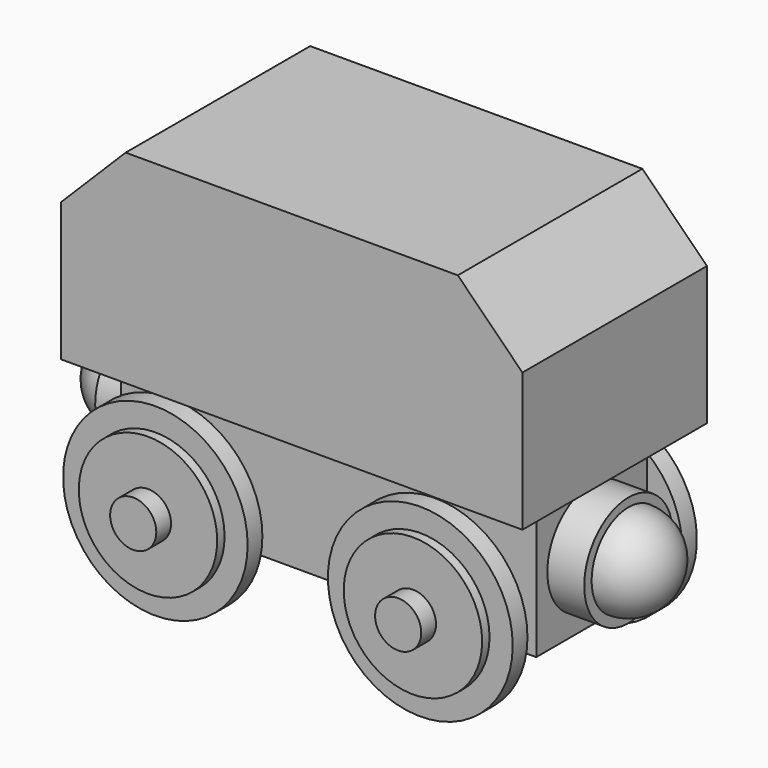
from build123d import *

# Parameters (mm, degrees)
F0_W      = 50
F0_H      = 22
F1_DEPTH  = 12.5
F2_W      = 45
F2_H      = 15
F3_DEPTH  = 15
F4_R      = 2.5
F5_DEPTH  = 3
F6_R      = 2.5
F7_DEPTH  = 3
F8_R      = 2.5
F9_DEPTH  = 3
F10_R     = 2.5
F11_DEPTH = 3
F12_R     = 10
F13_DEPTH = 2
F14_R     = 10
F15_DEPTH = 2
F16_R     = 10
F17_DEPTH = 2
F18_R     = 10.0146932226
F19_DEPTH = 2
F20_R     = 7.5
F21_DEPTH = 1
F22_R     = 7.5
F23_DEPTH = 1
F24_R     = 7.5
F25_DEPTH = 1
F26_R     = 7.3021705666
F27_DEPTH = 1
F28_R     = 2.5
F29_DEPTH = 2
F30_R     = 2.5
F31_DEPTH = 2
F32_R     = 2.5
F33_DEPTH = 2
F34_R     = 2.5
F35_DEPTH = 2
F36_R     = 6
F37_DEPTH = 4
F38_R     = 6
F39_DEPTH = 4
F42_SIZE  = 7
F43_SIZE  = 7


# Not quite as in the source:
# - a pattern or mirror of a feature is missing from the dataset's text; its kind, count and spacing are read off the source's solid


with BuildPart() as f1:
    # F0 (on Front) → F1 (new body, symmetric)
    with BuildSketch(Plane.XZ):
        Rectangle(F0_W, F0_H)
    extrude(amount=F1_DEPTH, both=True)

    # F2 (on face) → F3 (join)
    with BuildSketch(Plane(origin=(0, 0, -11), x_dir=(1, 0, 0), z_dir=(0, 0, -1))):
        Rectangle(F2_W, F2_H)
    extrude(amount=F3_DEPTH)

    # F4 (on face) → F5 (join)
    with BuildSketch(Plane.XZ.offset(7.5)):
        with Locations((13.9349065721, -22.4036108702)):
            Circle(F4_R)
    extrude(amount=F5_DEPTH)

    # F6 (on face) → F7 (join)
    with BuildSketch(Plane.XZ.offset(7.5)):
        with Locations((-14.7780319676, -22.1367031336)):
            Circle(F6_R)
    extrude(amount=F7_DEPTH)

    # F8 (on face) → F9 (join)
    with BuildSketch(Plane(origin=(0, 7.5, 0), x_dir=(-1, 0, 0), z_dir=(0, 1, 0))):
        with Locations((14.7414254025, -22.1880879253)):
            Circle(F8_R)
    extrude(amount=F9_DEPTH)

    # F10 (on face) → F11 (join)
    with BuildSketch(Plane(origin=(0, 7.5, 0), x_dir=(-1, 0, 0), z_dir=(0, 1, 0))):
        with Locations((-13.9084318653, -22.4365219474)):
            Circle(F10_R)
    extrude(amount=F11_DEPTH)

    # F12 (on face) → F13 (join)
    with BuildSketch(Plane(origin=(0, 10.5, 0), x_dir=(-1, 0, 0), z_dir=(0, 1, 0))):
        with Locations((-13.9084318653, -22.4365219474)):
            Circle(F12_R)
    extrude(amount=F13_DEPTH)

    # F14 (on face) → F15 (join)
    with BuildSketch(Plane(origin=(0, 10.5, 0), x_dir=(-1, 0, 0), z_dir=(0, 1, 0))):
        with Locations((14.7414254025, -22.1880879253)):
            Circle(F14_R)
    extrude(amount=F15_DEPTH)

    # F16 (on face) → F17 (join)
    with BuildSketch(Plane.XZ.offset(10.5)):
        with Locations((-14.7780319676, -22.1367031336)):
            Circle(F16_R)
    extrude(amount=F17_DEPTH)

    # F18 (on face) → F19 (join)
    with BuildSketch(Plane.XZ.offset(10.5)):
        with Locations((13.9349065721, -22.4036108702)):
            Circle(F18_R)
    extrude(amount=F19_DEPTH)

    # F20 (on face) → F21 (join)
    with BuildSketch(Plane.XZ.offset(12.5)):
        with Locations((-14.7780319676, -22.1367031336)):
            Circle(F20_R)
    extrude(amount=F21_DEPTH)

    # F22 (on face) → F23 (join)
    with BuildSketch(Plane.XZ.offset(12.5)):
        with Locations((13.9349065721, -22.4036108702)):
            Circle(F22_R)
    extrude(amount=F23_DEPTH)

    # F24 (on face) → F25 (join)
    with BuildSketch(Plane(origin=(0, 12.5, 0), x_dir=(-1, 0, 0), z_dir=(0, 1, 0))):
        with Locations((-13.9084318653, -22.4365219474)):
            Circle(F24_R)
    extrude(amount=F25_DEPTH)

    # F26 (on face) → F27 (join)
    with BuildSketch(Plane(origin=(0, 12.5, 0), x_dir=(-1, 0, 0), z_dir=(0, 1, 0))):
        with Locations((14.7414254025, -22.1880879253)):
            Circle(F26_R)
    extrude(amount=F27_DEPTH)

    # F28 (on face) → F29 (join)
    with BuildSketch(Plane(origin=(0, 13.5, 0), x_dir=(-1, 0, 0), z_dir=(0, 1, 0))):
        with Locations((-13.9084318653, -22.4365219474)):
            Circle(F28_R)
    extrude(amount=F29_DEPTH)

    # F30 (on face) → F31 (join)
    with BuildSketch(Plane(origin=(0, 13.5, 0), x_dir=(-1, 0, 0), z_dir=(0, 1, 0))):
        with Locations((14.7414254025, -22.1880879253)):
            Circle(F30_R)
    extrude(amount=F31_DEPTH)

    # F32 (on face) → F33 (join)
    with BuildSketch(Plane.XZ.offset(13.5)):
        with Locations((-14.7780319676, -22.1367031336)):
            Circle(F32_R)
    extrude(amount=F33_DEPTH)

    # F34 (on face) → F35 (join)
    with BuildSketch(Plane.XZ.offset(13.5)):
        with Locations((13.9349065721, -22.4036108702)):
            Circle(F34_R)
    extrude(amount=F35_DEPTH)

    # F36 (on face) → F37 (join)
    with BuildSketch(Plane(origin=(-22.5, 0, 0), x_dir=(0, -1, 0), z_dir=(-1, 0, 0))):
        with Locations((0, -18.4352861294)):
            Circle(F36_R)
    extrude(amount=F37_DEPTH)

    # F38 (on face) → F39 (join)
    with BuildSketch(Plane.YZ.offset(22.5)):
        with Locations((0, -18.4992050543)):
            Circle(F38_R)
    extrude(amount=F39_DEPTH)

    # F40 (on face) → F41 (revolve)
    with BuildSketch(Plane(origin=(-26.5, 0, 0), x_dir=(0, -1, 0), z_dir=(-1, 0, 0))):
        with BuildLine():
            Line((0, -23.4352861294), (0, -13.4352861294))
            ThreePointArc((0, -13.4352861294), (-5, -18.4352861294), (0, -23.4352861294))
        make_face()
    f41 = revolve(axis=Axis((-26.5, 0, -18.4352861294), (0, 0, -1)))

    # F41_copies: F41 across plane
    add(f41.mirror(Plane(origin=(0, 0, 0), x_dir=(0, 0, 1), z_dir=(1, 0, 0))))

    # F42
    f42_edges = [f1.edges().sort_by_distance(p)[0] for p in [
        (-25, 0, 11),
    ]]
    chamfer(f42_edges, length=F42_SIZE)

    # F43
    f43_edges = [f1.edges().sort_by_distance(p)[0] for p in [
        (25, 0, 11),
    ]]
    chamfer(f43_edges, length=F43_SIZE)


solid = f1.part
